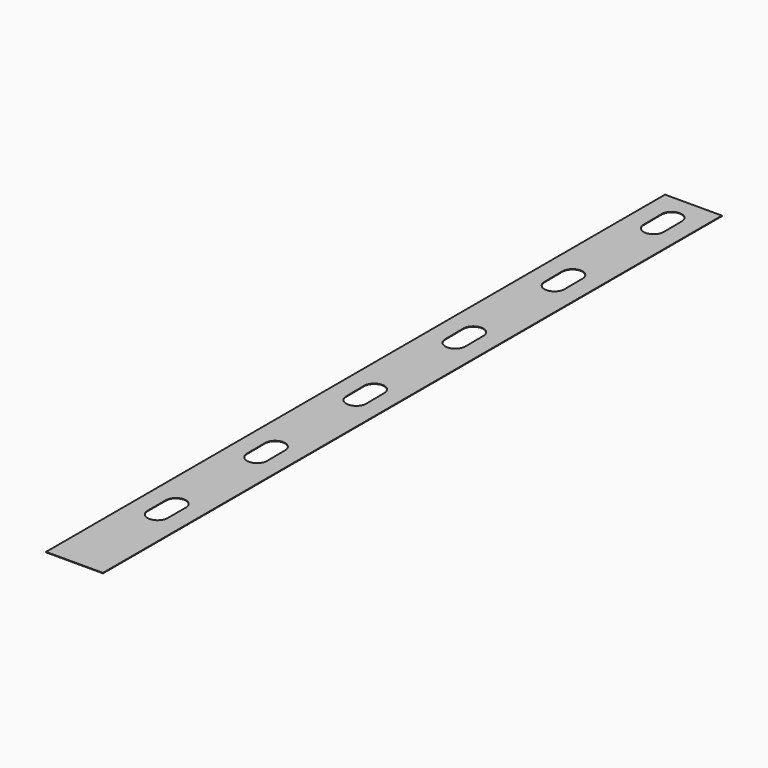
from build123d import *

# Parameters (mm, degrees)
F0_W     = 75
F0_H     = 1020
F1_DEPTH = 0.65


# Not quite as in the source:
# - ends of sketch curves that miss each other by under 0.0002 mm in the source are joined


with BuildPart() as f1:
    # F0 (on Top) → F1 (new body)
    with BuildSketch(Plane.XY):
        with Locations((-126.3066948975, -59.6911867905)):
            Rectangle(F0_W, F0_H)
        with BuildLine():
            ThreePointArc((-113.1066948975, -432.6711867905), (-126.3066948975, -445.8711867905), (-139.5066948975, -432.6711867905))
            Line((-139.5066948975, -432.6711867905), (-139.5066948975, -402.6711867905))
            ThreePointArc((-139.5066948975, -402.6711867905), (-126.3066948975, -389.4711867905), (-113.1066948975, -402.6711867905))
            Line((-113.1066948975, -402.6711867905), (-113.1066948975, -432.6711867905))
        make_face(mode=Mode.SUBTRACT)
        with BuildLine():
            ThreePointArc((-139.5059699251, -239.411547845), (-126.4450377578, -226.0739299572), (-113.10741987, -239.1348621245))
            Line((-113.10741987, -239.1348621245), (-112.7930042784, -269.1332144598))
            ThreePointArc((-112.7930042784, -269.1332144598), (-125.8539364457, -282.4708323476), (-139.1915543335, -269.4099001804))
            Line((-139.1915543335, -269.4099001804), (-139.5059699251, -239.411547845))
        make_face(mode=Mode.SUBTRACT)
        with BuildLine():
            ThreePointArc((-139.5059629442, -76.0142499203), (-126.4457022055, -62.6759745657), (-113.1074268508, -75.7362353044))
            Line((-113.1074268508, -75.7362353044), (-112.7915011509, -105.7345717742))
            ThreePointArc((-112.7915011509, -105.7345717742), (-125.8517618897, -119.0728471288), (-139.1900372443, -106.0125863901))
            Line((-139.1900372443, -106.0125863901), (-139.5059629442, -76.0142499203))
        make_face(mode=Mode.SUBTRACT)
        with BuildLine():
            ThreePointArc((-139.505960843, 87.3835072291), (-126.4459015791, 100.7219798561), (-113.107428952, 87.6619205922))
            Line((-113.107428952, 87.6619205922), (-112.7910501303, 57.6635888979))
            ThreePointArc((-112.7910501303, 57.6635888979), (-125.8511093943, 44.3251162708), (-139.1895820213, 57.3851755348))
            Line((-139.1895820213, 57.3851755348), (-139.505960843, 87.3835072291))
        make_face(mode=Mode.SUBTRACT)
        with BuildLine():
            ThreePointArc((-139.5062126227, 250.8085359622), (-126.4195302765, 264.1208890664), (-113.1071771723, 251.0342067202))
            Line((-113.1071771723, 251.0342067202), (-112.8507331291, 221.0353027993))
            ThreePointArc((-112.8507331291, 221.0353027993), (-125.9374154753, 207.7229496952), (-139.2497685795, 220.8096320413))
            Line((-139.2497685795, 220.8096320413), (-139.5062126227, 250.8085359622))
        make_face(mode=Mode.SUBTRACT)
        with BuildLine():
            ThreePointArc((-139.5060659261, 414.1907621397), (-126.4355531533, 427.5189914241), (-113.1073238689, 414.4484786514))
            Line((-113.1073238689, 414.4484786514), (-112.8144641966, 384.4499081319))
            ThreePointArc((-112.8144641966, 384.4499081319), (-125.8849769693, 371.1216788475), (-139.2132062537, 384.1921916203))
            Line((-139.2132062537, 384.1921916203), (-139.5060659261, 414.1907621397))
        make_face(mode=Mode.SUBTRACT)
    extrude(amount=F1_DEPTH)


solid = f1.part
